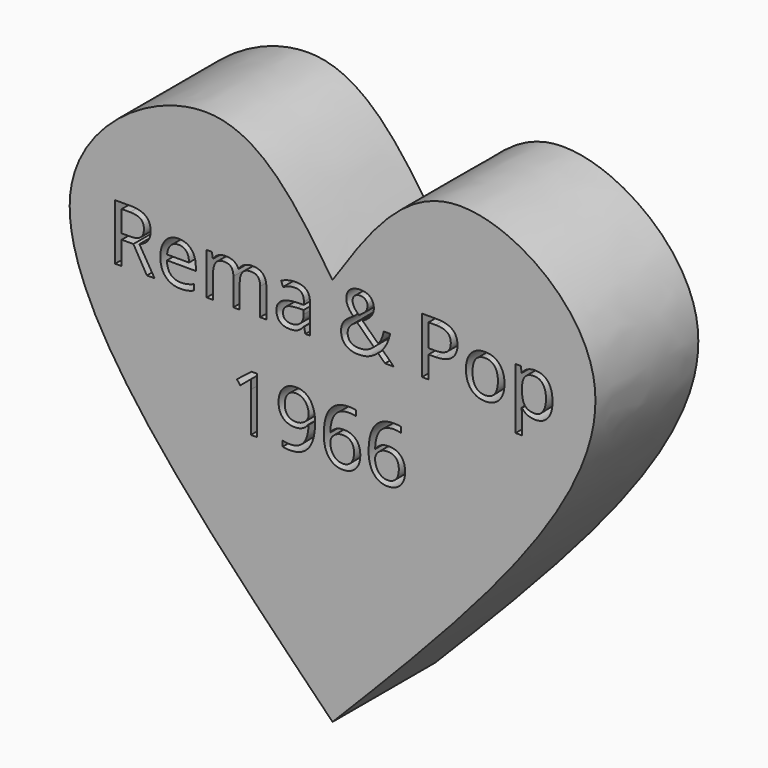
from build123d import *

# Parameters (mm, degrees)
F1_DEPTH     = 12.7
F2_TEXT_SIZE = 7.7394781946
F3_DEPTH     = 25.4


# Not quite as in the source:
# - Text() gives the source's letters only with a copy of the font that has no kerning and outlines rounded to 1/6400 em; it was checked with that copy


with BuildPart() as f1:
    # F0 (on Front) → F1 (new body)
    with BuildSketch(Plane.XZ):
        with BuildLine():
            add(Edge.make_bspline(
                [(0, 0), (3.410529145, 5.0602821755), (10.3835197518, 15.4062720725), (36.3007981473, -1.4677452915), (13.8949242386, -24.2769921546), (0, -38.4220667183)],
                knots=[0, 0, 0, 0, 0.266675861, 0.5452316033, 1, 1, 1, 1], degree=3))
            add(Edge.make_bspline(
                [(0, 0), (-3.410529145, 5.0602821755), (-10.3835197518, 15.4062720725), (-36.3007981473, -1.4677452915), (-13.8949242386, -24.2769921546), (0, -38.4220667183)],
                knots=[0, 0, 0, 0, 0.266675861, 0.5452316033, 1, 1, 1, 1], degree=3))
        make_face()
    extrude(amount=F1_DEPTH)

    # F2 (on face) → F3 (cut)
    with BuildSketch(Plane.XZ.offset(12.7)):
        with Locations((-22.225, -5.5724243001)):
            Text('Rema & Pop', F2_TEXT_SIZE, font='Open Sans', text_align=(TextAlign.LEFT, TextAlign.BOTTOM))
        with Locations((-10.1586697772, -16.0981146448)):
            Text('1966', F2_TEXT_SIZE, font='Open Sans', text_align=(TextAlign.LEFT, TextAlign.BOTTOM))
    extrude(amount=-F3_DEPTH, mode=Mode.SUBTRACT)


solid = f1.part
